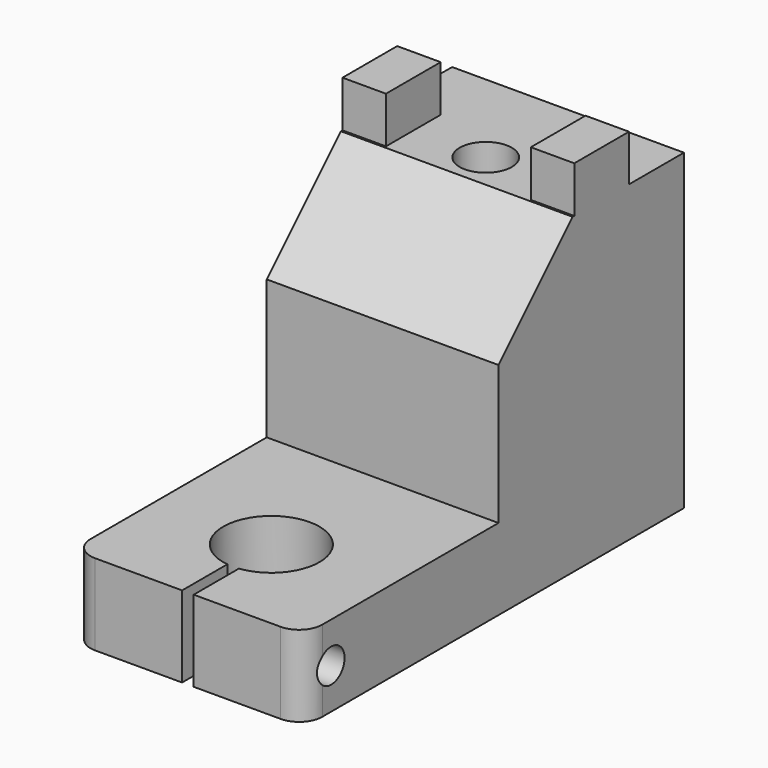
from build123d import *

# Parameters (mm, degrees)
F1_DEPTH    = 7
F2_R        = 1.45
F3_DEPTH    = 25
F4_T1_DEPTH = 17
F5_DEPTH    = 27
F0_W        = 3.75
F0_H        = 5.9
F6_DEPTH    = 31
F7_SIZE     = 8


# Not quite as in the source:
# - a fillet or chamfer that OpenCascade refuses, or shapes differently, is made with other operations: its cross-section is extruded or revolved along the edge and cut away or added


with BuildPart() as f1:
    # F0 (on Top) → F1 (new body)
    with BuildSketch(Plane.XY):
        with BuildLine():
            Line((-6.5963959517, 29.175), (-6.5963959517, 21))
            Line((-6.5963959517, 21), (3.4036040483, 21))
            Line((3.4036040483, 21), (3.4036040483, 29.875))
            ThreePointArc((3.4036040483, 29.875), (1.8126137907, 30.5340097423), (1.1536040483, 32.125))
            ThreePointArc((1.1536040483, 32.125), (1.8126137907, 33.7159902577), (3.4036040483, 34.375))
            Line((3.4036040483, 34.375), (3.4036040483, 41))
            Line((3.4036040483, 41), (-6.5963959517, 41))
            Line((-6.5963959517, 41), (-6.5963959517, 35.075))
            Line((-6.5963959517, 35.075), (-2.8463959517, 35.075))
            Line((-2.8463959517, 35.075), (-2.8463959517, 29.175))
            Line((-2.8463959517, 29.175), (-6.5963959517, 29.175))
        make_face()
        with BuildLine():
            Line((3.4036040483, 29.875), (3.4036040483, 21))
            Line((3.4036040483, 21), (13.4036040483, 21))
            Line((13.4036040483, 21), (13.4036040483, 29.175))
            Line((13.4036040483, 29.175), (9.6536040483, 29.175))
            Line((9.6536040483, 29.175), (9.6536040483, 35.075))
            Line((9.6536040483, 35.075), (13.4036040483, 35.075))
            Line((13.4036040483, 35.075), (13.4036040483, 41))
            Line((13.4036040483, 41), (3.4036040483, 41))
            Line((3.4036040483, 41), (3.4036040483, 34.375))
            ThreePointArc((3.4036040483, 34.375), (4.994594306, 33.7159902577), (5.6536040483, 32.125))
            ThreePointArc((5.6536040483, 32.125), (4.994594306, 30.5340097423), (3.4036040483, 29.875))
        make_face()
        with BuildLine():
            Line((-6.5963959517, 21), (-6.5963959517, 0))
            Line((-6.5963959517, 0), (2.9036040483, 0))
            Line((2.9036040483, 0), (2.9036040483, 1.2661458509))
            ThreePointArc((2.9036040483, 1.2661458509), (-1.8967497135, 14.6540914389), (11.1536040483, 9))
            ThreePointArc((11.1536040483, 9), (9.0576954873, 3.6996462382), (3.9036040483, 1.2661458509))
            Line((3.9036040483, 1.2661458509), (3.9036040483, 0))
            Line((3.9036040483, 0), (13.4036040483, 0))
            Line((13.4036040483, 0), (13.4036040483, 21))
            Line((13.4036040483, 21), (3.4036040483, 21))
            Line((3.4036040483, 21), (-6.5963959517, 21))
        make_face()
        with BuildLine():
            ThreePointArc((11.1536040483, 9), (-1.8967497135, 14.6540914389), (2.9036040483, 1.2661458509))
            Line((2.9036040483, 1.2661458509), (2.9036040483, 4.880230589))
            ThreePointArc((2.9036040483, 4.880230589), (0.6515593539, 12.1062437123), (7.5536040483, 9))
            ThreePointArc((7.5536040483, 9), (6.5098477606, 6.2479553056), (3.9036040483, 4.880230589))
            Line((3.9036040483, 4.880230589), (3.9036040483, 1.2661458509))
            ThreePointArc((3.9036040483, 1.2661458509), (9.0576954873, 3.6996462382), (11.1536040483, 9))
        make_face()
    extrude(amount=F1_DEPTH)

    # F2 (on face) → F3 (cut)
    with BuildSketch(Plane.YZ.offset(13.4036040483)):
        with Locations((2.95, 3.5)):
            Circle(F2_R)
    extrude(amount=-F3_DEPTH, mode=Mode.SUBTRACT)

    # F4: fillet of radius 2 on 2 edges, made by hand

    # F4_s2 → F4_t1 (cut)
    with BuildSketch(Plane.XY.offset(-5)):
        with BuildLine():
            ThreePointArc((11.4036040483, 0), (12.8178176107, 0.5857864376), (13.4036040483, 2))
            Line((13.4036040483, 2), (13.4036040483, 0))
            Line((13.4036040483, 0), (11.4036040483, 0))
        make_face()
        with BuildLine():
            ThreePointArc((-6.5963959517, 2), (-6.010609514, 0.5857864376), (-4.5963959517, 0))
            Line((-4.5963959517, 0), (-6.5963959517, 0))
            Line((-6.5963959517, 0), (-6.5963959517, 2))
        make_face()
    extrude(amount=F4_T1_DEPTH, mode=Mode.SUBTRACT)

    # F0 (on Top) → F5 (join)
    with BuildSketch(Plane.XY):
        with BuildLine():
            Line((3.4036040483, 29.875), (3.4036040483, 21))
            Line((3.4036040483, 21), (13.4036040483, 21))
            Line((13.4036040483, 21), (13.4036040483, 29.175))
            Line((13.4036040483, 29.175), (9.6536040483, 29.175))
            Line((9.6536040483, 29.175), (9.6536040483, 35.075))
            Line((9.6536040483, 35.075), (13.4036040483, 35.075))
            Line((13.4036040483, 35.075), (13.4036040483, 41))
            Line((13.4036040483, 41), (3.4036040483, 41))
            Line((3.4036040483, 41), (3.4036040483, 34.375))
            ThreePointArc((3.4036040483, 34.375), (4.994594306, 33.7159902577), (5.6536040483, 32.125))
            ThreePointArc((5.6536040483, 32.125), (4.994594306, 30.5340097423), (3.4036040483, 29.875))
        make_face()
        with BuildLine():
            Line((-6.5963959517, 29.175), (-6.5963959517, 21))
            Line((-6.5963959517, 21), (3.4036040483, 21))
            Line((3.4036040483, 21), (3.4036040483, 29.875))
            ThreePointArc((3.4036040483, 29.875), (1.8126137907, 30.5340097423), (1.1536040483, 32.125))
            ThreePointArc((1.1536040483, 32.125), (1.8126137907, 33.7159902577), (3.4036040483, 34.375))
            Line((3.4036040483, 34.375), (3.4036040483, 41))
            Line((3.4036040483, 41), (-6.5963959517, 41))
            Line((-6.5963959517, 41), (-6.5963959517, 35.075))
            Line((-6.5963959517, 35.075), (-2.8463959517, 35.075))
            Line((-2.8463959517, 35.075), (-2.8463959517, 29.175))
            Line((-2.8463959517, 29.175), (-6.5963959517, 29.175))
        make_face()
    extrude(amount=F5_DEPTH)

    # F0 (on Top) → F6 (join)
    with BuildSketch(Plane.XY):
        with Locations((-4.7213959517, 32.125)):
            Rectangle(F0_W, F0_H)
        with Locations((11.5286040483, 32.125)):
            Rectangle(F0_W, F0_H)
    extrude(amount=F6_DEPTH)

    # F7
    f7_edges = [f1.edges().sort_by_distance(p)[0] for p in [
        (3.403604, 21, 27),
    ]]
    chamfer(f7_edges, length=F7_SIZE)


solid = f1.part
